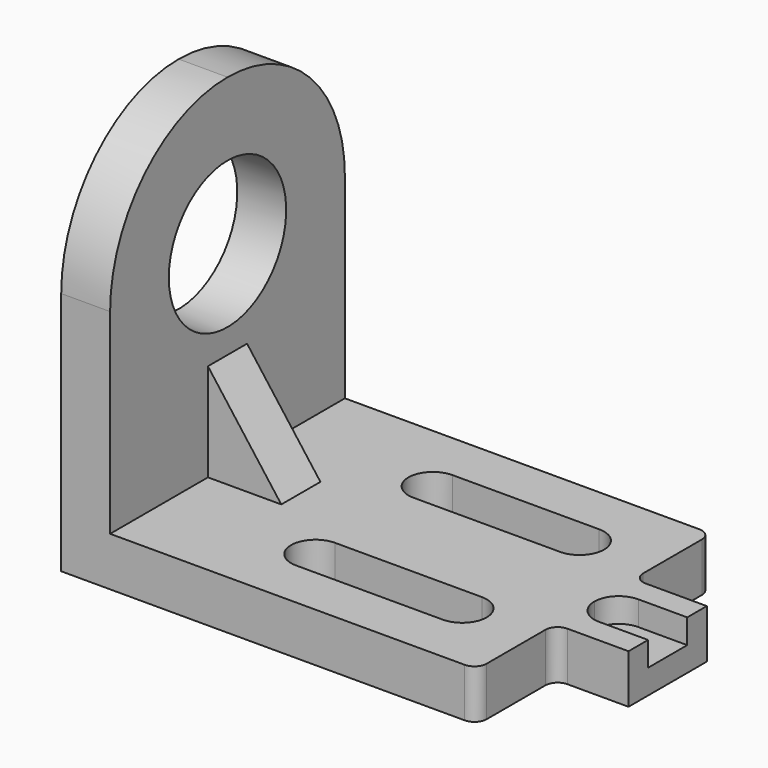
from build123d import *

# Parameters (mm, degrees)
F1_DEPTH = 12.7
F2_DEPTH = 12.7
F3_R     = 38.1
F4_DEPTH = 25.4
F6_START = -63.5
F6_DEPTH = 25.4


with BuildPart() as f1:
    # F0 (on Top) → F1 (new body, symmetric)
    with BuildSketch(Plane.XY):
        with BuildLine():
            Line((0, 152.4), (0, 0))
            Line((0, 0), (101.6, 0))
            Line((101.6, 0), (209.55, 0))
            ThreePointArc((209.55, 0), (214.040128, 1.859872), (215.9, 6.35))
            Line((215.9, 6.35), (215.9, 44.45))
            ThreePointArc((215.9, 44.45), (217.759872, 48.940128), (222.25, 50.8))
            Line((222.25, 50.8), (254, 50.8))
            Line((254, 50.8), (254, 63.5))
            Line((254, 63.5), (228.6, 63.5))
            ThreePointArc((228.6, 63.5), (219.619744, 67.219744), (215.9, 76.2))
            ThreePointArc((215.9, 76.2), (219.619744, 85.180256), (228.6, 88.9))
            Line((228.6, 88.9), (254, 88.9))
            Line((254, 88.9), (254, 101.6))
            Line((254, 101.6), (222.25, 101.6))
            ThreePointArc((222.25, 101.6), (217.759872, 103.459872), (215.9, 107.95))
            Line((215.9, 107.95), (215.9, 146.05))
            ThreePointArc((215.9, 146.05), (214.040128, 150.540128), (209.55, 152.4))
            Line((209.55, 152.4), (101.6, 152.4))
            Line((101.6, 152.4), (0, 152.4))
        make_face()
        with BuildLine():
            Line((177.8, 25.4), (101.6, 25.4))
            ThreePointArc((101.6, 25.4), (88.9, 38.1), (101.6, 50.8))
            Line((101.6, 50.8), (177.8, 50.8))
            ThreePointArc((177.8, 50.8), (186.780256, 47.080256), (190.5, 38.1))
            ThreePointArc((190.5, 38.1), (186.780256, 29.119744), (177.8, 25.4))
        make_face(mode=Mode.SUBTRACT)
        with BuildLine():
            ThreePointArc((101.6, 101.6), (88.9, 114.3), (101.6, 127))
            Line((101.6, 127), (177.8, 127))
            ThreePointArc((177.8, 127), (186.780256, 123.280256), (190.5, 114.3))
            ThreePointArc((190.5, 114.3), (186.780256, 105.319744), (177.8, 101.6))
            Line((177.8, 101.6), (101.6, 101.6))
        make_face(mode=Mode.SUBTRACT)
    extrude(amount=F1_DEPTH, both=True)

    # F0 (on Top) → F2 (join)
    with BuildSketch(Plane.XY):
        with BuildLine():
            Line((228.6, 63.5), (254, 63.5))
            Line((254, 63.5), (254, 88.9))
            Line((254, 88.9), (228.6, 88.9))
            ThreePointArc((228.6, 88.9), (219.619744, 85.180256), (215.9, 76.2))
            ThreePointArc((215.9, 76.2), (219.619744, 67.219744), (228.6, 63.5))
        make_face()
    extrude(amount=-F2_DEPTH)

    # F3 (on face) → F4 (join)
    with BuildSketch(Plane(origin=(0, 0, 0), x_dir=(0, -1, 0), z_dir=(-1, 0, 0))):
        with BuildLine():
            Line((-152.4, 12.7), (0, 12.7))
            Line((0, 12.7), (0, 114.3))
            ThreePointArc((0, 114.3), (-22.318463, 168.181537), (-76.2, 190.5))
            ThreePointArc((-76.2, 190.5), (-130.081537, 168.181537), (-152.4, 114.3))
            Line((-152.4, 114.3), (-152.4, 12.7))
        make_face()
        with Locations((-76.2, 114.3)):
            Circle(F3_R, mode=Mode.SUBTRACT)
    extrude(amount=-F4_DEPTH)

    # F5 (on face) → F6 (join)
    with BuildSketch(Plane.XZ.offset(F6_START)):
        Polygon((25.4, 63.5), (25.4, 12.7), (63.5, 12.7), align=None)
    extrude(amount=-F6_DEPTH)


solid = f1.part
